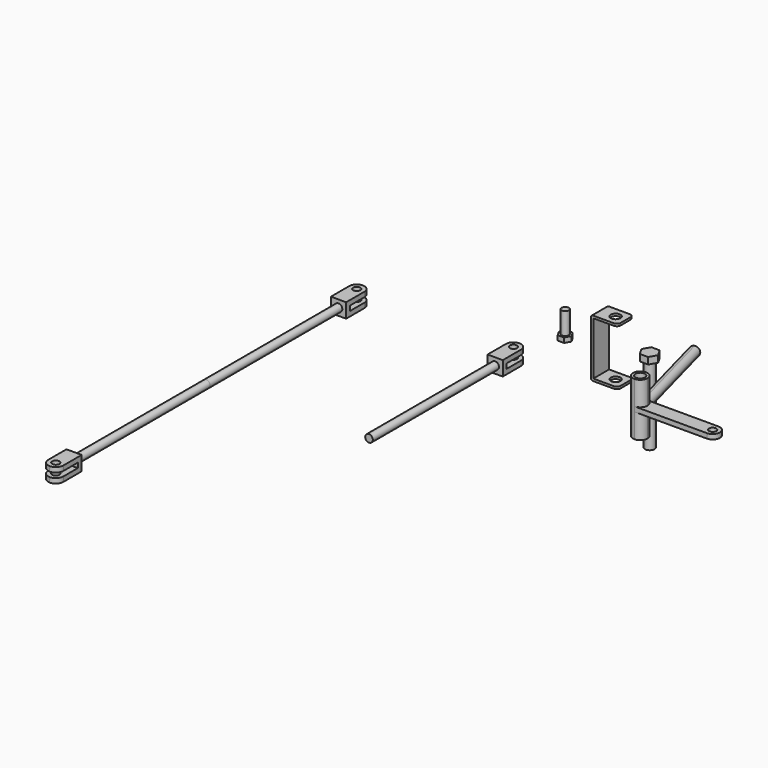
from build123d import *

# Parameters (mm, degrees)
F0_R          = 6.35
F0_W          = 3
F0_H          = 26
F1_DEPTH      = 3
F2_DEPTH      = 34.925
F5_DEPTH      = 8.73125
F6_R          = 6.35
F7_DEPTH      = 101.6
F8_R          = 6.35
F9_DEPTH      = 34.925
F10_R         = 2.5
F8_R_2        = 4.7625
F11_DEPTH     = 3.175
F12_DEPTH     = 6.35
F13_T4_DEPTH  = 157.7514773719
F13_T9_DEPTH  = 156.5536421667
F13_S10_R     = 9.525
F13_T11_DEPTH = 81
F13_T15_DEPTH = 157.7514773719
F13_T20_DEPTH = 156.5536421667
F13_S21_R     = 9.525
F13_T22_DEPTH = 81
F14_R         = 4.7625
F14_W         = 20
F14_H         = 6.35
F15_DEPTH     = 6.35
F16_DEPTH     = 3.175
F18_R         = 4.7625
F19_DEPTH     = 6.35
F20_DEPTH     = 35
F22_R         = 5
F23_DEPTH     = 217.3477245
F25_R         = 5
F26_DEPTH     = 207.3477245


# Not quite as in the source:
# - a fillet or chamfer that OpenCascade refuses, or shapes differently, is made with other operations: its cross-section is extruded or revolved along the edge and cut away or added


with BuildPart() as f1:
    # F0 (on Top) → F1 (new body)
    with BuildSketch(Plane.XY):
        with BuildLine():
            ThreePointArc((13, 8), (11.5355339059, 11.5355339059), (8, 13))
            Line((8, 13), (-19, 13))
            Line((-19, 13), (-19, -13))
            Line((-19, -13), (8, -13))
            ThreePointArc((8, -13), (11.5355339059, -11.5355339059), (13, -8))
            Line((13, -8), (13, 8))
        make_face()
        Circle(F0_R, mode=Mode.SUBTRACT)
        with Locations((-20.5, 0)):
            Rectangle(F0_W, F0_H)
    extrude(amount=-F1_DEPTH)

    # F0 (on Top) → F2 (join)
    with BuildSketch(Plane.XY):
        with Locations((-20.5, 0)):
            Rectangle(F0_W, F0_H)
    extrude(amount=F2_DEPTH)

    # F3: F1 across face


with BuildPart() as f1_1:
    add(f1.part)
    add(f1.part.mirror(Plane(origin=(-20.5, 0, 34.925), x_dir=(1, 0, 0), z_dir=(0, 0, 1))))

    # F10
    f10_edges = [f1_1.edges().sort_by_distance(p)[0] for p in [
        (-22, 0, 72.85),
        (-22, 0, -3),
    ]]
    fillet(f10_edges, radius=F10_R)


with BuildPart() as f5:
    # F4 (on Top) → F5 (new body)
    with BuildSketch(Plane.XY):
        Polygon((5.499261314, 65.5749876738), (-5.499261314, 65.5749876738), (-10.9985226281, 56.0499876738), (-5.499261314, 46.5249876738), (5.499261314, 46.5249876738), (10.9985226281, 56.0499876738), align=None)
    extrude(amount=F5_DEPTH)

    # F6 (on face) → F7 (join)
    with BuildSketch(Plane(origin=(0, 0, 0), x_dir=(1, 0, 0), z_dir=(0, 0, -1))):
        with Locations((0, -56.0499876738)):
            Circle(F6_R)
    extrude(amount=F7_DEPTH)


with BuildPart() as f9:
    # F8 (on Top) → F9 (new body, symmetric)
    with BuildSketch(Plane.XY):
        with BuildLine():
            ThreePointArc((56.427881222, -39.6455373057), (63.1630733128, -36.8557293965), (65.952881222, -30.1205373057))
            ThreePointArc((65.952881222, -30.1205373057), (63.1630733128, -23.3853452149), (56.427881222, -20.5955373057))
            ThreePointArc((56.427881222, -20.5955373057), (53.2429104438, -21.1438126167), (50.4246044097, -22.7255192182))
            ThreePointArc((50.4246044097, -22.7255192182), (47.451156533, -33.3055080839), (56.427881222, -39.6455373057))
        make_face()
        with Locations((56.427881222, -30.1205373057)):
            Circle(F8_R, mode=Mode.SUBTRACT)
    extrude(amount=F9_DEPTH, both=True)

    # F8 (on Top) → F11 (join, symmetric)
    with BuildSketch(Plane.XY):
        with BuildLine():
            ThreePointArc((56.427881222, -20.5955373057), (63.1630733128, -23.3853452149), (65.952881222, -30.1205373057))
            ThreePointArc((65.952881222, -30.1205373057), (63.1630733128, -36.8557293965), (56.427881222, -39.6455373057))
            Line((56.427881222, -39.6455373057), (151.676961222, -39.6455373057))
            ThreePointArc((151.676961222, -39.6455373057), (158.4121533128, -36.8557293965), (161.201961222, -30.1205373057))
            ThreePointArc((161.201961222, -30.1205373057), (158.4121533128, -23.3853452149), (151.676961222, -20.5955373057))
            Line((151.676961222, -20.5955373057), (63.0018849676, -20.5955373057))
            Line((63.0018849676, -20.5955373057), (56.427881222, -20.5955373057))
        make_face()
        with Locations((151.676961222, -30.1205373057)):
            Circle(F8_R_2, mode=Mode.SUBTRACT)
    extrude(amount=F11_DEPTH, both=True)

    # F8 (on Top) → F12 (join, symmetric)
    with BuildSketch(Plane.XY):
        with BuildLine():
            ThreePointArc((50.4246044097, -22.7255192182), (53.2429104438, -21.1438126167), (56.427881222, -20.5955373057))
            Line((56.427881222, -20.5955373057), (63.0018849676, -20.5955373057))
            Line((63.0018849676, -20.5955373057), (30.3903029127, 101.1125438384))
            Line((30.3903029127, 101.1125438384), (24.2566739158, 99.469042902))
            Line((24.2566739158, 99.469042902), (18.1230449188, 97.8255419656))
            Line((18.1230449188, 97.8255419656), (50.4246044097, -22.7255192182))
        make_face()
    extrude(amount=F12_DEPTH, both=True)

    # F13: fillet of radius 6.35 on 4 edges, made by hand


with BuildPart() as f13_tool2:
    # F13_s3 → F13_t4 (new body)
    with BuildSketch(Plane(origin=(13.4779627171, -50.3004416428, 0), x_dir=(0, 0, 1), z_dir=(-0.2588190451, 0.9659258263, 0))):
        with BuildLine():
            ThreePointArc((0, 55.5246304963), (4.4901280605, 53.6647585568), (6.35, 49.1746304963))
            Line((6.35, 49.1746304963), (6.35, 55.5246304963))
            Line((6.35, 55.5246304963), (0, 55.5246304963))
        make_face()
    extrude(amount=F13_T4_DEPTH)

    split(bisect_by=Plane.XZ.offset(20.5955373057), keep=Keep.BOTTOM)


with BuildPart() as f9_1:
    add(f9.part)

    # F13_t1: cut F13_tool2
    add(f13_tool2.part, mode=Mode.SUBTRACT)


with BuildPart() as f13_tool7:
    # F13_s8 → F13_t9 (new body)
    with BuildSketch(Plane(origin=(-27.3511240198, 102.075784486, 0), x_dir=(0, 0, 1), z_dir=(0.2588190451, -0.9659258263, 0))):
        with BuildLine():
            ThreePointArc((0, -42.8246304963), (4.4901280605, -44.6845024357), (6.35, -49.1746304963))
            Line((6.35, -49.1746304963), (6.35, -42.8246304963))
            Line((6.35, -42.8246304963), (0, -42.8246304963))
        make_face()
    extrude(amount=F13_T9_DEPTH)

    # F13_s10 → F13_t11 (cut, symmetric)
    with BuildSketch(Plane.XY.offset(3.2)):
        with Locations((56.427881222, -30.1205373057)):
            Circle(F13_S10_R)
    extrude(amount=F13_T11_DEPTH, both=True, mode=Mode.SUBTRACT)


with BuildPart() as f9_2:
    add(f9_1.part)

    # F13_t6: cut F13_tool7
    add(f13_tool7.part, mode=Mode.SUBTRACT)


with BuildPart() as f13_tool13:
    # F13_s14 → F13_t15 (new body)
    with BuildSketch(Plane(origin=(13.4779627171, -50.3004416428, 0), x_dir=(0, 0, 1), z_dir=(-0.2588190451, 0.9659258263, 0))):
        with BuildLine():
            ThreePointArc((0, 55.5246304963), (-4.4901280605, 53.6647585568), (-6.35, 49.1746304963))
            Line((-6.35, 49.1746304963), (-6.35, 55.5246304963))
            Line((-6.35, 55.5246304963), (0, 55.5246304963))
        make_face()
    extrude(amount=F13_T15_DEPTH)

    split(bisect_by=Plane.XZ.offset(20.5955373057), keep=Keep.BOTTOM)


with BuildPart() as f9_3:
    add(f9_2.part)

    # F13_t12: cut F13_tool13
    add(f13_tool13.part, mode=Mode.SUBTRACT)


with BuildPart() as f13_tool18:
    # F13_s19 → F13_t20 (new body)
    with BuildSketch(Plane(origin=(-27.3511240198, 102.075784486, 0), x_dir=(0, 0, 1), z_dir=(0.2588190451, -0.9659258263, 0))):
        with BuildLine():
            ThreePointArc((0, -42.8246304963), (-4.4901280605, -44.6845024357), (-6.35, -49.1746304963))
            Line((-6.35, -49.1746304963), (-6.35, -42.8246304963))
            Line((-6.35, -42.8246304963), (0, -42.8246304963))
        make_face()
    extrude(amount=F13_T20_DEPTH)

    # F13_s21 → F13_t22 (cut, symmetric)
    with BuildSketch(Plane.XY.offset(-3.2)):
        with Locations((56.427881222, -30.1205373057)):
            Circle(F13_S21_R)
    extrude(amount=F13_T22_DEPTH, both=True, mode=Mode.SUBTRACT)


with BuildPart() as f9_4:
    add(f9_3.part)

    # F13_t17: cut F13_tool18
    add(f13_tool18.part, mode=Mode.SUBTRACT)


with BuildPart() as f15:
    # F14 (on Top) → F15 (new body)
    with BuildSketch(Plane.XY):
        with BuildLine():
            Line((-121.9479370444, -51.7426801049), (-101.9479370444, -51.7426801049))
            Line((-101.9479370444, -51.7426801049), (-101.9479370444, -28.0926801049))
            ThreePointArc((-101.9479370444, -28.0926801049), (-104.8768692325, -21.021612293), (-111.9479370444, -18.0926801049))
            ThreePointArc((-111.9479370444, -18.0926801049), (-119.0190048563, -21.021612293), (-121.9479370444, -28.0926801049))
            Line((-121.9479370444, -28.0926801049), (-121.9479370444, -51.7426801049))
        make_face()
        with Locations((-111.9479370444, -28.0926801049)):
            Circle(F14_R, mode=Mode.SUBTRACT)
        with Locations((-111.9479370444, -54.9176801049)):
            Rectangle(F14_W, F14_H)
    extrude(amount=-F15_DEPTH)

    # F14 (on Top) → F16 (join)
    with BuildSketch(Plane.XY):
        with Locations((-111.9479370444, -54.9176801049)):
            Rectangle(F14_W, F14_H)
    extrude(amount=F16_DEPTH)

    # F17: F15 across face


with BuildPart() as f15_1:
    add(f15.part)
    add(f15.part.mirror(Plane(origin=(-111.9479370444, -54.9176801049, 3.175), x_dir=(1, 0, 0), z_dir=(0, 0, 1))))


with BuildPart() as f19:
    # F18 (on Top) → F19 (new body)
    with BuildSketch(Plane.XY):
        Polygon((-91.9003056777, 44.2796825945), (-100.1491976487, 44.2796825945), (-104.2736436343, 37.1359325945), (-100.1491976487, 29.9921825945), (-91.9003056777, 29.9921825945), (-87.7758596922, 37.1359325945), align=None)
        with Locations((-96.0247516632, 37.1359325945)):
            Circle(F18_R, mode=Mode.SUBTRACT)
        with Locations((-96.0247516632, 37.1359325945)):
            Circle(F18_R)
    extrude(amount=F19_DEPTH)

    # F18 (on Top) → F20 (join)
    with BuildSketch(Plane.XY):
        with Locations((-96.0247516632, 37.1359325945)):
            Circle(F18_R)
    extrude(amount=F20_DEPTH)


with BuildPart() as f21_1:
    # F21: copy of F15
    add(f15_1.part.moved(Location((-206, 0, 0))))

    # F22 (on face) → F23 (join)
    with BuildSketch(Plane.XZ.offset(58.0926801049)):
        with Locations((-317.9479370444, 3.175)):
            Circle(F22_R)
    extrude(amount=F23_DEPTH)

    # F24: F21_1 across face


with BuildPart() as f21_1_1:
    add(f21_1.part)
    add(f21_1.part.mirror(Plane(origin=(-317.9479370444, -275.4404046049, 3.175), x_dir=(1, 0, 0), z_dir=(0, -1, 0))))


with BuildPart() as f15_2:
    add(f15_1.part)

    # F25 (on face) → F26 (join)
    with BuildSketch(Plane.XZ.offset(58.0926801049)):
        with Locations((-111.9479370444, 3.175)):
            Circle(F25_R)
    extrude(amount=F26_DEPTH)


solid = Compound([f1_1.part, f5.part, f9_4.part, f19.part, f21_1_1.part, f15_2.part])
